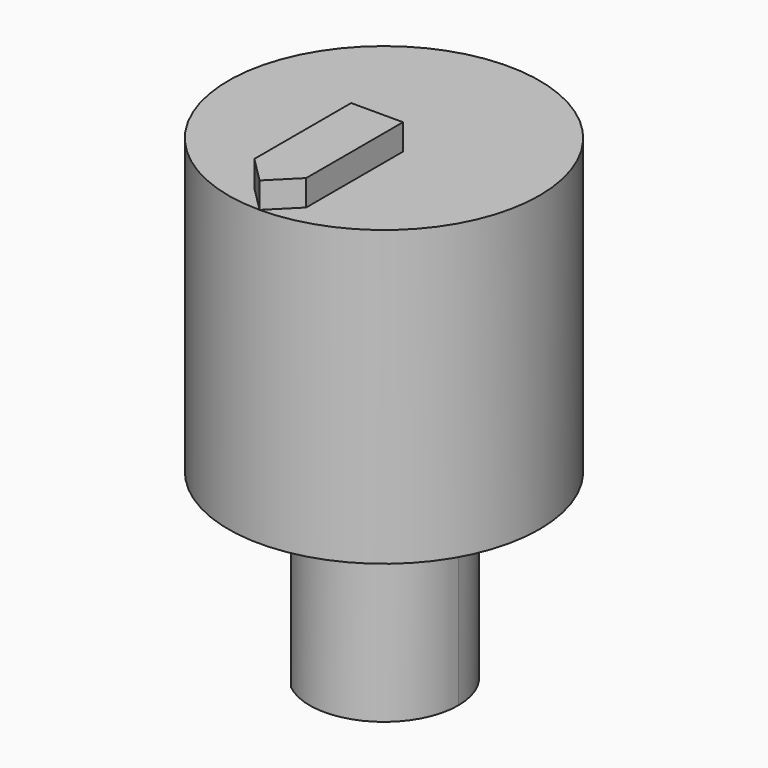
from build123d import *

# Parameters (mm, degrees)
F0_R     = 9
F1_DEPTH = 17
F2_DEPTH = 10.5
F4_DEPTH = 1.5


# Not quite as in the source:
# - a feature names something its author has since deleted; it is built from what else it names


with BuildPart() as f1:
    # F0 (on Top) → F1 (new body)
    with BuildSketch(Plane.XY):
        Circle(F0_R)
        with BuildLine():
            ThreePointArc((-2.7, 3.3466401061), (1.8547236991, 3.8794329483), (4.3, 0))
            ThreePointArc((4.3, 0), (1.8547236991, -3.8794329483), (-2.7, -3.3466401061))
            ThreePointArc((-2.7, -3.3466401061), (-4.3, 0), (-2.7, 3.3466401061))
        make_face(mode=Mode.SUBTRACT)
        with BuildLine():
            ThreePointArc((-2.7, -3.3466401061), (1.8547236991, -3.8794329483), (4.3, 0))
            ThreePointArc((4.3, 0), (1.8547236991, 3.8794329483), (-2.7, 3.3466401061))
            Line((-2.7, 3.3466401061), (-2.7, -3.3466401061))
        make_face()
        with BuildLine():
            Line((-1.7, -2.8284271247), (-1.7, 2.8284271247))
            ThreePointArc((-1.7, 2.8284271247), (3.3, 0), (-1.7, -2.8284271247))
        make_face(mode=Mode.SUBTRACT)
        with BuildLine():
            ThreePointArc((-1.7, -2.8284271247), (3.3, 0), (-1.7, 2.8284271247))
            Line((-1.7, 2.8284271247), (-1.7, -2.8284271247))
        make_face()
        with BuildLine():
            Line((-2.7, -3.3466401061), (-2.7, 3.3466401061))
            ThreePointArc((-2.7, 3.3466401061), (-4.3, 0), (-2.7, -3.3466401061))
        make_face()
    extrude(amount=F1_DEPTH)

    # F0 (on Top) → F2 (join)
    with BuildSketch(Plane.XY):
        with BuildLine():
            ThreePointArc((-2.7, -3.3466401061), (1.8547236991, -3.8794329483), (4.3, 0))
            ThreePointArc((4.3, 0), (1.8547236991, 3.8794329483), (-2.7, 3.3466401061))
            Line((-2.7, 3.3466401061), (-2.7, -3.3466401061))
        make_face()
        with BuildLine():
            Line((-1.7, -2.8284271247), (-1.7, 2.8284271247))
            ThreePointArc((-1.7, 2.8284271247), (3.3, 0), (-1.7, -2.8284271247))
        make_face(mode=Mode.SUBTRACT)
    extrude(amount=-F2_DEPTH)

    # F3 (on face) → F4 (join)
    with BuildSketch(Plane.XY.offset(17)):
        Polygon((-1.5, -7.5), (0, -9), (1.5, -7.5), (1.5, -0.5), (-1.5, -0.5), align=None)
    extrude(amount=F4_DEPTH)


solid = f1.part
